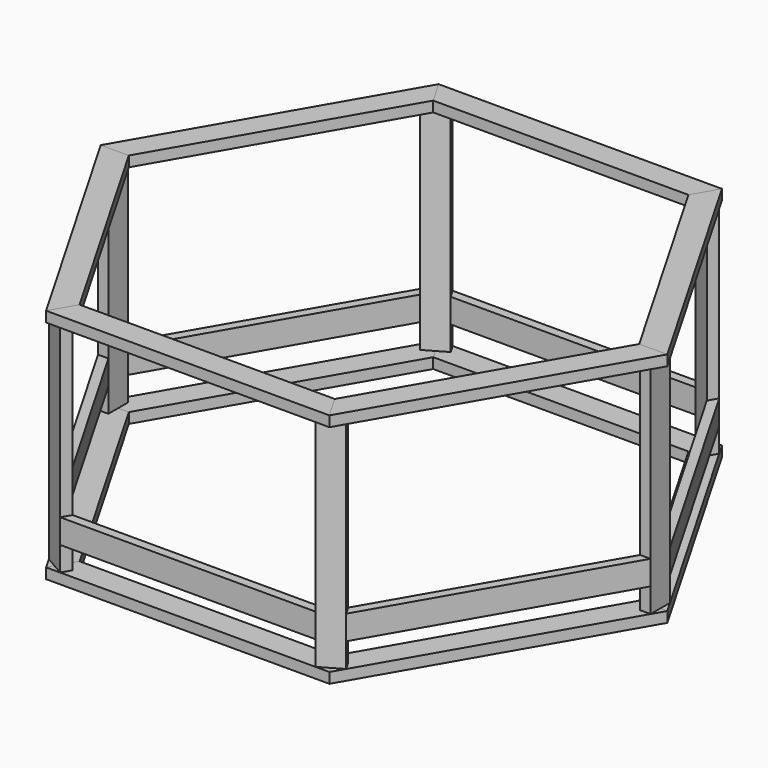
from build123d import *

# Parameters (mm, degrees)
F5_DEPTH  = 38.1
F6_DEPTH  = 38.1
F7_DEPTH  = 38.1
F8_DEPTH  = 38.1
F9_DEPTH  = 38.1
F10_DEPTH = 38.1
F11_W     = 38.1
F11_H     = 44.45
F12_DEPTH = 787.4
F13_DEPTH = 787.4
F14_DEPTH = 787.4
F11_H_2   = 88.9
F15_DEPTH = 787.4
F16_DEPTH = 787.4
F17_DEPTH = 787.4
F18_DEPTH = 88.9
F19_DEPTH = 88.9
F20_DEPTH = 88.9
F21_DEPTH = 88.9
F22_DEPTH = 88.9
F23_DEPTH = 88.9


# Not quite as in the source:
# - a variable given as a bare number and used for a length is read in inches; the dataset says mm whatever the document's units were


with BuildPart() as f5:
    # F4 (on Top) → F5 (new body)
    with BuildSketch(Plane.XY):
        Polygon((-466.2640359457, 807.593), (-517.5904748766, 896.493), (-1035.1809497532, 0), (-932.5280718913, 0), align=None)
    extrude(amount=F5_DEPTH)


with BuildPart() as f6:
    # F4 (on Top) → F6 (new body)
    with BuildSketch(Plane.XY):
        Polygon((517.5904748766, 896.493), (-517.5904748766, 896.493), (-466.2640359457, 807.593), (466.2640359457, 807.593), align=None)
    extrude(amount=F6_DEPTH)


with BuildPart() as f7:
    # F4 (on Top) → F7 (new body)
    with BuildSketch(Plane.XY):
        Polygon((1035.1809497532, 0), (517.5904748766, 896.493), (466.2640359457, 807.593), (932.5280718913, 0), align=None)
    extrude(amount=F7_DEPTH)


with BuildPart() as f8:
    # F4 (on Top) → F8 (new body)
    with BuildSketch(Plane.XY):
        Polygon((517.5904748766, -896.493), (1035.1809497532, 0), (932.5280718913, 0), (466.2640359457, -807.593), align=None)
    extrude(amount=F8_DEPTH)


with BuildPart() as f9:
    # F4 (on Top) → F9 (new body)
    with BuildSketch(Plane.XY):
        Polygon((-466.2640359457, -807.593), (-517.5904748766, -896.493), (517.5904748766, -896.493), (466.2640359457, -807.593), align=None)
    extrude(amount=F9_DEPTH)


with BuildPart() as f10:
    # F4 (on Top) → F10 (new body)
    with BuildSketch(Plane.XY):
        Polygon((-932.5280718913, 0), (-1035.1809497532, 0), (-517.5904748766, -896.493), (-466.2640359457, -807.593), align=None)
    extrude(amount=F10_DEPTH)


with BuildPart() as f12:
    # F11 (on face) → F12 (new body)
    with BuildSketch(Plane.XY.offset(38.1)):
        with Locations((-990.4677302878, 22.225)):
            Rectangle(F11_W, F11_H)
        with Locations((-990.4677302878, -22.225)):
            Rectangle(F11_W, F11_H)
    extrude(amount=F12_DEPTH)


with BuildPart() as f13:
    # F11 (on face) → F13 (new body)
    with BuildSketch(Plane.XY.offset(38.1)):
        Polygon((-504.7588651439, 874.268), (-543.2536943421, 852.043), (-524.2036943421, 819.0474321158), (-485.7088651439, 841.2724321158), align=None)
        Polygon((-466.2640359457, 896.493), (-504.7588651439, 874.268), (-485.7088651439, 841.2724321158), (-447.2140359457, 863.4974321158), align=None)
    extrude(amount=F13_DEPTH)


with BuildPart() as f14:
    # F11 (on face) → F14 (new body)
    with BuildSketch(Plane.XY.offset(38.1)):
        Polygon((543.2536943421, 852.043), (466.2640359457, 896.493), (447.2140359457, 863.4974321158), (524.2036943421, 819.0474321158), align=None)
    extrude(amount=F14_DEPTH)


with BuildPart() as f15:
    # F11 (on face) → F15 (new body)
    with BuildSketch(Plane.XY.offset(38.1)):
        with Locations((990.4677302878, 0)):
            Rectangle(F11_W, F11_H_2)
    extrude(amount=F15_DEPTH)


with BuildPart() as f16:
    # F11 (on face) → F16 (new body)
    with BuildSketch(Plane.XY.offset(38.1)):
        Polygon((447.2140359457, -863.4974321158), (466.2640359457, -896.493), (543.2536943421, -852.043), (524.2036943421, -819.0474321158), align=None)
    extrude(amount=F16_DEPTH)


with BuildPart() as f17:
    # F11 (on face) → F17 (new body)
    with BuildSketch(Plane.XY.offset(38.1)):
        Polygon((-524.2036943421, -819.0474321158), (-543.2536943421, -852.043), (-466.2640359457, -896.493), (-447.2140359457, -863.4974321158), align=None)
    extrude(amount=F17_DEPTH)


with BuildPart() as f18:
    # F11 (on face) → F18 (new body)
    with BuildSketch(Plane.XY.offset(38.1)):
        Polygon((-447.2140359457, -863.4974321158), (-466.2640359457, -896.493), (466.2640359457, -896.493), (447.2140359457, -863.4974321158), align=None)
    extrude(amount=F18_DEPTH)


with BuildPart() as f19:
    # F11 (on face) → F19 (new body)
    with BuildSketch(Plane.XY.offset(38.1)):
        Polygon((524.2036943421, -819.0474321158), (543.2536943421, -852.043), (1009.5177302878, -44.45), (971.4177302878, -44.45), align=None)
    extrude(amount=F19_DEPTH)


with BuildPart() as f20:
    # F11 (on face) → F20 (new body)
    with BuildSketch(Plane.XY.offset(38.1)):
        Polygon((1009.5177302878, 44.45), (543.2536943421, 852.043), (524.2036943421, 819.0474321158), (971.4177302878, 44.45), align=None)
    extrude(amount=F20_DEPTH)


with BuildPart() as f21:
    # F11 (on face) → F21 (new body)
    with BuildSketch(Plane.XY.offset(38.1)):
        Polygon((466.2640359457, 896.493), (-466.2640359457, 896.493), (-447.2140359457, 863.4974321158), (447.2140359457, 863.4974321158), align=None)
    extrude(amount=F21_DEPTH)


with BuildPart() as f22:
    # F11 (on face) → F22 (new body)
    with BuildSketch(Plane.XY.offset(38.1)):
        Polygon((-543.2536943421, 852.043), (-1009.5177302878, 44.45), (-971.4177302878, 44.45), (-524.2036943421, 819.0474321158), align=None)
    extrude(amount=F22_DEPTH)


with BuildPart() as f23:
    # F11 (on face) → F23 (new body)
    with BuildSketch(Plane.XY.offset(38.1)):
        Polygon((-971.4177302878, -44.45), (-1009.5177302878, -44.45), (-543.2536943421, -852.043), (-524.2036943421, -819.0474321158), align=None)
    extrude(amount=F23_DEPTH)


with BuildPart() as f23_1:
    # F24: moved
    add(f23.part.moved(Location((0, 0, 88.9))))


with BuildPart() as f22_1:
    # F24: moved
    add(f22.part.moved(Location((0, 0, 88.9))))


with BuildPart() as f21_1:
    # F24: moved
    add(f21.part.moved(Location((0, 0, 88.9))))


with BuildPart() as f20_1:
    # F24: moved
    add(f20.part.moved(Location((0, 0, 88.9))))


with BuildPart() as f19_1:
    # F24: moved
    add(f19.part.moved(Location((0, 0, 88.9))))


with BuildPart() as f18_1:
    # F24: moved
    add(f18.part.moved(Location((0, 0, 88.9))))


with BuildPart() as f25_1:
    # F25: copy of F5
    add(f5.part.moved(Location((0, 0, 825.5))))


with BuildPart() as f25_2:
    # F25: copy of F6
    add(f6.part.moved(Location((0, 0, 825.5))))


with BuildPart() as f25_3:
    # F25: copy of F7
    add(f7.part.moved(Location((0, 0, 825.5))))


with BuildPart() as f25_4:
    # F25: copy of F8
    add(f8.part.moved(Location((0, 0, 825.5))))


with BuildPart() as f25_5:
    # F25: copy of F9
    add(f9.part.moved(Location((0, 0, 825.5))))


with BuildPart() as f25_6:
    # F25: copy of F10
    add(f10.part.moved(Location((0, 0, 825.5))))


solid = Compound([f5.part, f6.part, f7.part, f8.part, f9.part, f10.part, f12.part, f13.part, f14.part, f15.part, f16.part, f17.part, f23_1.part, f22_1.part, f21_1.part, f20_1.part, f19_1.part, f18_1.part, f25_1.part, f25_2.part, f25_3.part, f25_4.part, f25_5.part, f25_6.part])
